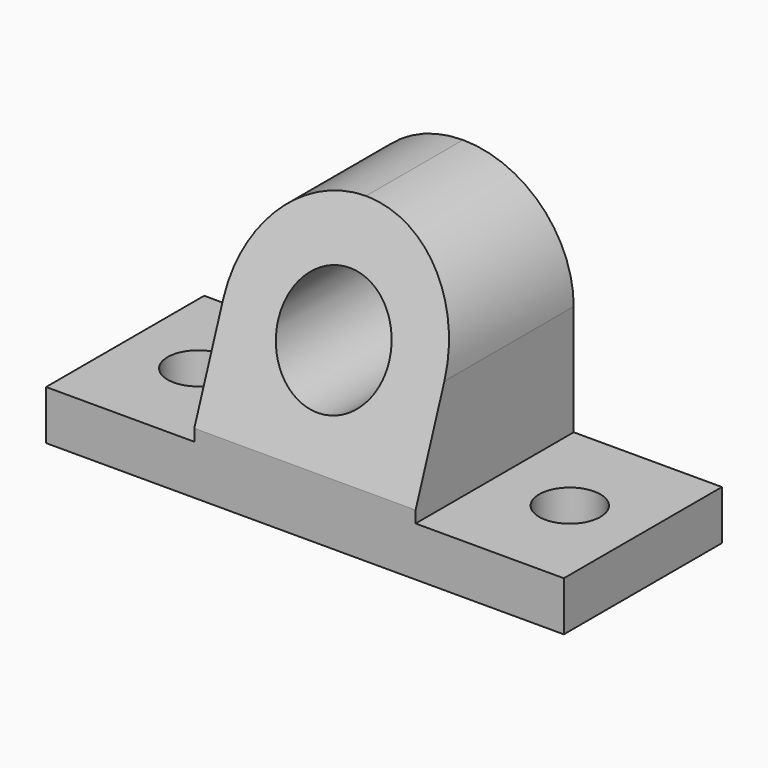
from build123d import *

# Parameters (mm, degrees)
F0_W      = 133.096
F0_H      = 50.8
F1_DEPTH  = 12.7
F2_W      = 56.896
F2_H      = 50.8
F3_DEPTH  = 56.896
F4_SIZE2  = 53.848
F4_SIZE   = 19.6088
F5_R      = 14.2875
F6_DEPTH  = 50.8
F7_R      = 28.44799
F9_R      = 7.874
F8_R      = 7.874
F10_DEPTH = 25.4


# Not quite as in the source:
# - a fillet or chamfer is up to 0.001 mm smaller than in the source, because OpenCascade refuses the exact size


with BuildPart() as f1:
    # F0 (on Top) → F1 (new body)
    with BuildSketch(Plane.XY):
        with Locations((66.548, -25.4)):
            Rectangle(F0_W, F0_H)
    extrude(amount=F1_DEPTH)

    # F2 (on face) → F3 (join)
    with BuildSketch(Plane.XY.offset(12.7)):
        with Locations((66.548, -25.4)):
            Rectangle(F2_W, F2_H)
    extrude(amount=F3_DEPTH)

    # F4
    f4_edges = [f1.edges().sort_by_distance(p)[0] for p in [
        (66.548, -50.8, 69.596),
    ]]
    f4_side = f1.faces().sort_by_distance((66.548, -25.4, 69.596))[0]
    chamfer(f4_edges, length=F4_SIZE, length2=F4_SIZE2, reference=f4_side)

    # F5 (on face) → F6 (cut)
    with BuildSketch(Plane(origin=(0, 0, 0), x_dir=(-1, 0, 0), z_dir=(0, 1, 0))):
        with Locations((-66.548, 41.148)):
            Circle(F5_R)
    extrude(amount=-F6_DEPTH, mode=Mode.SUBTRACT)

    # F7 (radius 28.448 in the source; OpenCascade refuses exactly that, so slightly less here)
    f7_edges = [f1.edges().sort_by_distance(p)[0] for p in [
        (94.996, -15.5956, 69.596),
        (38.1, -15.5956, 69.596),
    ]]
    fillet(f7_edges, radius=F7_R)

    # F9 (on face) + F8 (on face) → F10 (cut)
    with BuildSketch(Plane(origin=(0, 0, 0), x_dir=(1, 0, 0), z_dir=(0, 0, -1))):
        with Locations((18.796, 25.4)):
            Circle(F9_R)
    with BuildSketch(Plane(origin=(0, 0, 0), x_dir=(1, 0, 0), z_dir=(0, 0, -1))):
        with Locations((114.3, 25.4)):
            Circle(F8_R)
    extrude(amount=-F10_DEPTH, mode=Mode.SUBTRACT)


solid = f1.part
